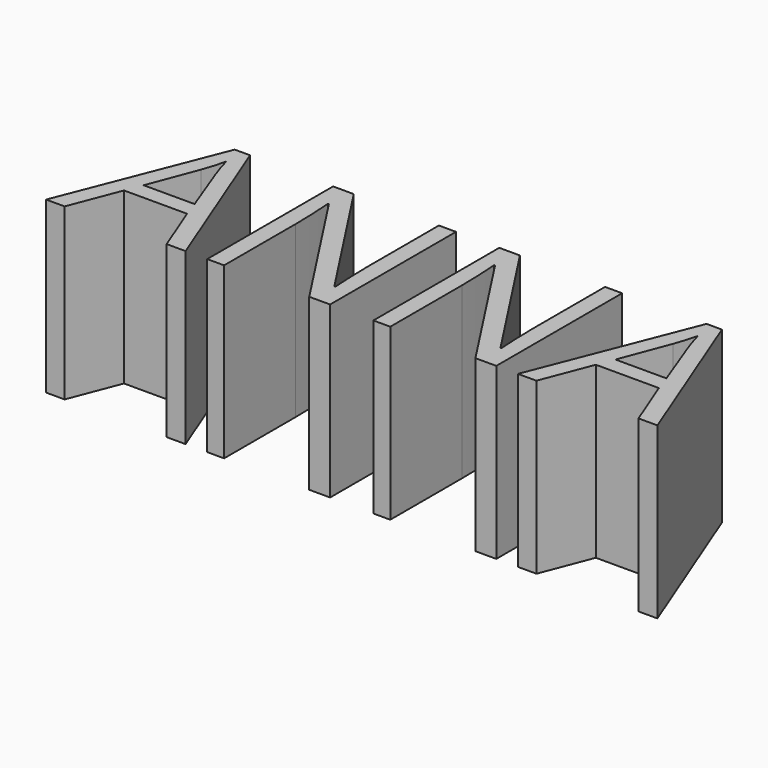
from build123d import *

# Parameters (mm, degrees)
F0_TEXT_SIZE = 98.8346834977
F1_DEPTH     = 76.2


# Not quite as in the source:
# - Text() gives the source's letters only with a copy of the font that has no kerning and outlines rounded to 1/6400 em; it was checked with that copy


with BuildPart() as f1:
    # F0 (on Top) → F1 (new body)
    with BuildSketch(Plane.XY):
        with Locations((-25.9018559009, -34.3821793795)):
            Text('ANNA', F0_TEXT_SIZE, font='Open Sans', text_align=(TextAlign.LEFT, TextAlign.BOTTOM))
    extrude(amount=F1_DEPTH)


solid = f1.part
